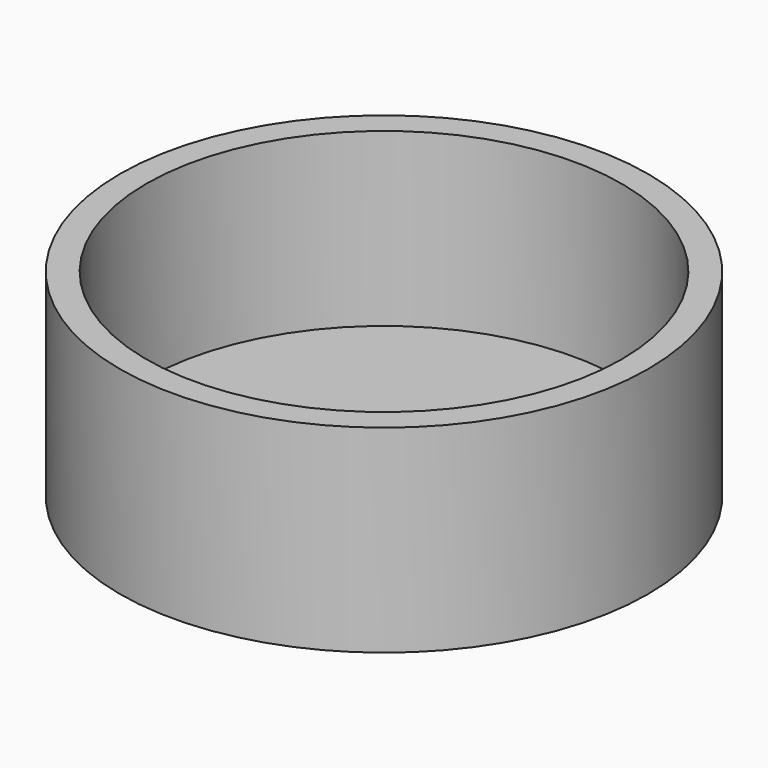
from build123d import *

# Parameters (mm, degrees)
F0_R     = 20
F1_DEPTH = 15
F2_R     = 18
F3_DEPTH = 13


# Not quite as in the source:
# - the program builds the solid bodies; features that only make, move or delete a surface that nothing else refers to are left out


with BuildPart() as f1:
    # F0 (on Top) → F1 (new body)
    with BuildSketch(Plane.XY):
        with Locations((0, -2.7690164279)):
            Circle(F0_R)
    extrude(amount=F1_DEPTH)

    # F2 (on face) → F3 (cut)
    with BuildSketch(Plane.XY.offset(15)):
        with Locations((0, -2.7690164279)):
            Circle(F2_R)
    extrude(amount=-F3_DEPTH, mode=Mode.SUBTRACT)


solid = f1.part
